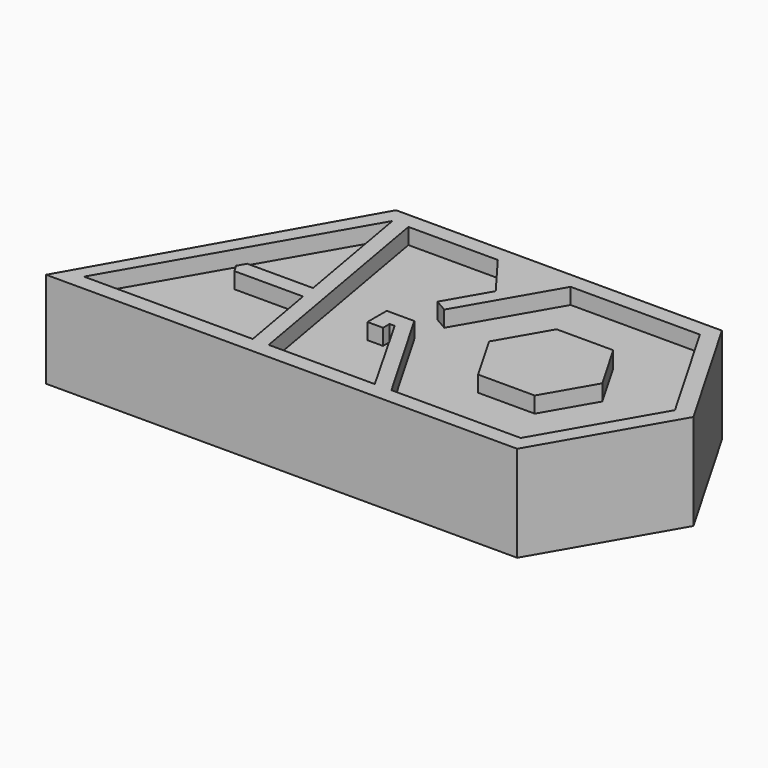
from build123d import *

# Parameters (mm, degrees)
F1_DEPTH      = 2
F2_DEPTH      = 10
F3_DEPTH      = 10
F5_R          = 4.5
F6_DEPTH      = 7.75
F7_R          = 3.017766953
F8_DEPTH      = 2
F8_DEPTH_BACK = 10


with BuildPart() as f1:
    # F0 (on Top) → F1 (new body)
    with BuildSketch(Plane.XY):
        Polygon((16.2767896806, 4.7439276241), (9.1951099779, 4.7439276241), (5.6542701265, -1.3889868999), (9.1951099779, -7.5219014239), (16.2767896806, -7.5219014239), (19.8176295319, -1.3889868999), align=None)
    extrude(amount=F1_DEPTH)



with BuildPart() as f1b:
    # F0 (on Top) → F1, piece 2 (new body)
    with BuildSketch(Plane.XY):
        Polygon((-17.6287352592, 14.6110131001), (-18.7731224283, 14.6110131001), (-36.9286165964, -17.3889868999), (-33.7945427965, -17.3889868999), (-12.6915797993, -17.3889868999), (-10.6915797993, -17.3889868999), (4.6530460606, -17.3889868999), (21.9735541363, -17.3889868999), (31.2111584433, -1.3889868999), (21.9735541363, 14.6110131001), (4.6530460606, 14.6110131001), (-15.6287352592, 14.6110131001), align=None)
        Polygon((-10.6915797993, -15.3889868999), (-15.6287352592, 12.6110131001), (-4.4508377103, 12.6110131001), (2.5694442447, 12.6110131001), (4.6530460606, 12.6110131001), (20.8188535979, 12.6110131001), (28.9017573665, -1.3889868999), (20.8188535979, -15.3889868999), (4.6530460606, -15.3889868999), (2.5684264704, -15.3889868999), align=None, mode=Mode.SUBTRACT)
        Polygon((-12.6915797993, -15.3889868999), (-33.7945427965, -15.3889868999), (-17.6287352592, 12.6110131001), (-14.8230012653, -3.3010950903), (-23.0469053902, -3.3010950903), (-23.6242556594, -4.3010950903), (-23.0469053902, -5.3010950903), (-14.4703473038, -5.3010950903), align=None, mode=Mode.SUBTRACT)
        Polygon((1.4286793875, -13.3889868999), (2.5684264704, -15.3889868999), (4.6530460606, -15.3889868999), (-2.7495239491, -2.5673595365), (-6.1911302619, -2.5673595365), (-6.1911302619, -5.5895005353), (-4.2386944406, -5.5895005353), (-4.2386944406, -4.5673595365), (-3.5985326394, -4.5673595365), align=None)
        Polygon((4.6530460606, 12.6110131001), (2.5694442447, 12.6110131001), (0.814373756, 9.5711418427), (-0.4812889005, 7.3269882922), (-3.5320220458, 2.0429634842), (-1.9693206839, 1.1407374323), align=None)
    extrude(amount=F1_DEPTH)


with BuildPart() as f1_1:
    add(f1.part)

    add(f1b.part)  # F2 merges F1b
    # F0 (on Top) → F2 (join)
    with BuildSketch(Plane.XY):
        Polygon((-17.6287352592, 12.6110131001), (-33.7945427965, -15.3889868999), (-12.6915797993, -15.3889868999), (-14.4703473038, -5.3010950903), (-23.0469053902, -5.3010950903), (-23.6242556594, -4.3010950903), (-23.0469053902, -3.3010950903), (-14.8230012653, -3.3010950903), align=None)
        Polygon((-4.4508377103, 12.6110131001), (-15.6287352592, 12.6110131001), (-10.6915797993, -15.3889868999), (2.5684264704, -15.3889868999), (1.4286793875, -13.3889868999), (-3.5985326394, -4.5673595365), (-4.2386944406, -4.5673595365), (-4.2386944406, -5.5895005353), (-6.1911302619, -5.5895005353), (-6.1911302619, -2.5673595365), (-2.7495239491, -2.5673595365), (4.6530460606, -15.3889868999), (20.8188535979, -15.3889868999), (28.9017573665, -1.3889868999), (20.8188535979, 12.6110131001), (4.6530460606, 12.6110131001), (-1.9693206839, 1.1407374323), (-3.5320220458, 2.0429634842), (-0.4812889005, 7.3269882922), align=None)
        Polygon((5.6542701265, -1.3889868999), (9.1951099779, 4.7439276241), (16.2767896806, 4.7439276241), (19.8176295319, -1.3889868999), (16.2767896806, -7.5219014239), (9.1951099779, -7.5219014239), align=None, mode=Mode.SUBTRACT)
    extrude(amount=-F2_DEPTH)

    # F3 (add): faces of the model
    f3_faces = [f1_1.faces().sort_by_distance(p)[0] for p in [
        (-3.8174957495, -2.6316950576, 0),
        (12.7359498292, -1.3889868999, 0),
    ]]
    extrude(f3_faces, amount=F3_DEPTH)

    # F4: union 

    # F5 (on face) → F6 (cut)
    with BuildSketch(Plane(origin=(0, 0, -10), x_dir=(1, 0, 0), z_dir=(0, 0, -1))):
        with Locations((12.7852637746, 0)):
            Circle(F5_R)
        with Locations((-8.9510052619, 0)):
            Circle(F5_R)
    extrude(amount=-F6_DEPTH, mode=Mode.SUBTRACT)

    # F7
    f7_edges = [f1_1.edges().sort_by_distance(p)[0] for p in [
        (8.285264, 0, -2.25),
        (-13.451005, 0, -2.25),
    ]]
    fillet(f7_edges, radius=F7_R)

    # F0 (on Top) → F8 (join, two sides)
    with BuildSketch(Plane.XY) as f8_sk:
        Polygon((0.814373756, 9.5711418427), (-4.4508377103, 12.6110131001), (-0.4812889005, 7.3269882922), align=None)
        Polygon((2.5694442447, 12.6110131001), (-4.4508377103, 12.6110131001), (0.814373756, 9.5711418427), align=None)
    extrude(amount=F8_DEPTH)
    extrude(f8_sk.sketch, amount=-F8_DEPTH_BACK)


with BuildPart() as f9_1:
    # F9: copy of F1
    add(f1_1.part)


solid = Compound([f1_1.part, f9_1.part])
